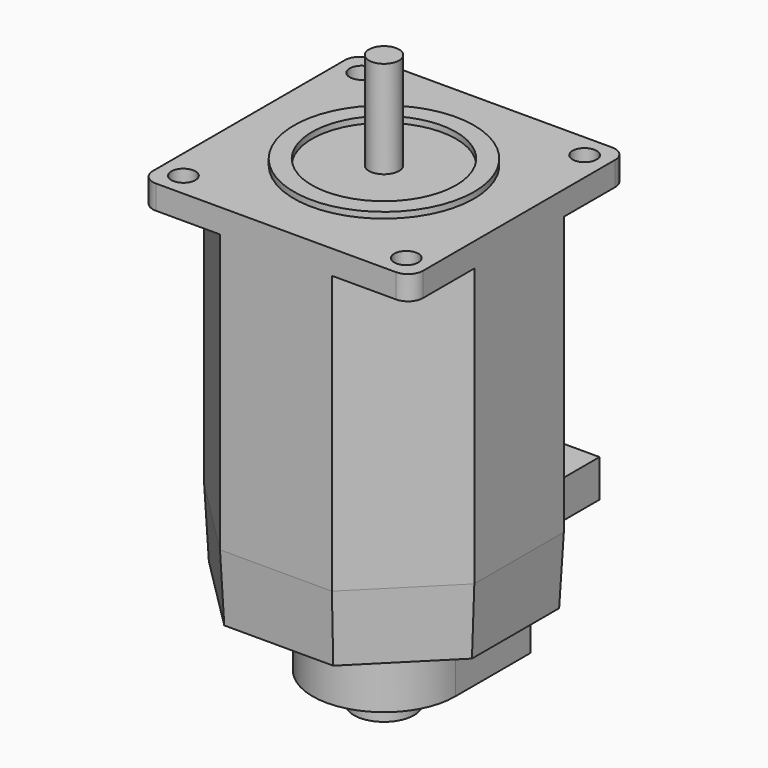
from build123d import *

# Parameters (mm, degrees)
F0_R                   = 2.54
F0_R_2                 = 19.05
F0_R_3                 = 15.24
F0_R_4                 = 3.175
F1_DEPTH               = 5.08
F2_DEPTH               = 1.27
F3_DEPTH               = 20.574
F5_DEPTH               = 58.7375
F6_DEPTH               = 14.2875
DRAFT_F6_DRAFTED_ANGLE = 3
F7_R                   = 6.35
F8_DEPTH               = 22.225
F9_DEPTH               = 15.875
F11_DEPTH              = 3.175
F12_DEPTH              = 12.7
F13_T                  = 1.27
F13_T3_DEPTH           = 26.2123050896
F13_T5_DEPTH           = 3.9232108179
F13_T7_DEPTH           = 10.4992710847
F13_T9_DEPTH           = 3.6795314226
F13_T11_DEPTH          = 26.0744592074
F13_T13_DEPTH          = 3.6795314226
F13_T15_DEPTH          = 10.4992710847
F13_T17_DEPTH          = 3.9232108179
F13_T19_DEPTH          = 26.2123050896
F13_T21_DEPTH          = 25.7298445017
F13_T23_DEPTH          = 22.38375
F13_T25_DEPTH          = 32.7025
F13_T27_DEPTH          = 26.2123050896
F13_T29_DEPTH          = 26.2123050896
F13_T34_ANGLE          = 180.000000001


# Not quite as in the source:
# - an extrude with a draft is written as a straight extrude whose walls are then drafted
# - a shell that OpenCascade refuses in one call is made with other operations: the cavity is built on its own and cut out


with BuildPart() as f1:
    # F0 (on Top) → F1 (new body)
    with BuildSketch(Plane.XY):
        with BuildLine():
            Line((-53.975, 0), (-3.175, 0))
            ThreePointArc((-3.175, 0), (-0.9299359697, 0.9299359697), (0, 3.175))
            Line((0, 3.175), (0, 53.975))
            ThreePointArc((0, 53.975), (-0.9299359697, 56.2200640303), (-3.175, 57.15))
            Line((-3.175, 57.15), (-53.975, 57.15))
            ThreePointArc((-53.975, 57.15), (-56.2200640303, 56.2200640303), (-57.15, 53.975))
            Line((-57.15, 53.975), (-57.15, 3.175))
            ThreePointArc((-57.15, 3.175), (-56.2200640303, 0.9299359697), (-53.975, 0))
        make_face()
        with Locations((-52.1481723178, 5.0018276822)):
            Circle(F0_R, mode=Mode.SUBTRACT)
        with Locations((-5.0018276822, 5.0018276822)):
            Circle(F0_R, mode=Mode.SUBTRACT)
        with Locations((-52.1481723178, 52.1481723178)):
            Circle(F0_R, mode=Mode.SUBTRACT)
        with Locations((-28.575, 28.575)):
            Circle(F0_R_2, mode=Mode.SUBTRACT)
        with Locations((-5.0018276822, 52.1481723178)):
            Circle(F0_R, mode=Mode.SUBTRACT)
        with Locations((-28.575, 28.575)):
            Circle(F0_R_2)
        with Locations((-28.575, 28.575)):
            Circle(F0_R_3, mode=Mode.SUBTRACT)
        with Locations((-28.575, 28.575)):
            Circle(F0_R_3)
        with Locations((-28.575, 28.575)):
            Circle(F0_R_4, mode=Mode.SUBTRACT)
        with Locations((-28.575, 28.575)):
            Circle(F0_R_4)
    extrude(amount=-F1_DEPTH)

    # F0 (on Top) → F2 (join)
    with BuildSketch(Plane.XY):
        with Locations((-28.575, 28.575)):
            Circle(F0_R_2)
        with Locations((-28.575, 28.575)):
            Circle(F0_R_3, mode=Mode.SUBTRACT)
    extrude(amount=F2_DEPTH)

    # F0 (on Top) → F3 (join)
    with BuildSketch(Plane.XY):
        with Locations((-28.575, 28.575)):
            Circle(F0_R_4)
    extrude(amount=F3_DEPTH)

    # F4 (on face) → F5 (join)
    with BuildSketch(Plane(origin=(0, 0, -5.08), x_dir=(1, 0, 0), z_dir=(0, 0, -1))):
        Polygon((-40.4111525448, -57.15), (-16.7388474552, -57.15), (0, -40.4111525448), (0, -16.7388474552), (-16.7388474552, 0), (-40.4111525448, 0), (-57.15, -16.7388474552), (-57.15, -40.4111525448), align=None)
    extrude(amount=F5_DEPTH)


with BuildPart() as f6_drafted:
    # F6 (new): a face of the model
    f6_faces = [f1.part.faces().sort_by_distance(p)[0] for p in [
        (-28.575, 28.575, -63.8175),
    ]]
    extrude(f6_faces, amount=F6_DEPTH)

    # draft_F6_drafted
    draft_f6_drafted_walls = [f6_drafted.faces().sort_by_distance(p)[0] for p in [
        (-28.575, 57.15, -73.3425),
        (-8.3694237276, 48.7805762724, -73.3425),
        (0, 28.575, -73.3425),
        (-8.3694237276, 8.3694237276, -73.3425),
        (-28.575, 0, -73.3425),
        (-48.7805762724, 8.3694237276, -73.3425),
        (-57.15, 28.575, -73.3425),
        (-48.7805762724, 48.7805762724, -73.3425),
    ]]
    draft(draft_f6_drafted_walls, neutral_plane=Plane(origin=(-28.575, 28.575, -63.8175), x_dir=(1, 0, 0), z_dir=(0, 0, -1)), angle=DRAFT_F6_DRAFTED_ANGLE)


with BuildPart() as f1_1:
    add(f1.part)

    # join_F6_drafted: union F6_drafted
    add(f6_drafted.part)

    # F7 (on face) → F8 (join)
    with BuildSketch(Plane(origin=(0, 0, -78.105), x_dir=(1, 0, 0), z_dir=(0, 0, -1))):
        with Locations((-28.575, -28.575)):
            Circle(F7_R)
    extrude(amount=F8_DEPTH)

    # F7 (on face) → F9 (join)
    with BuildSketch(Plane(origin=(0, 0, -78.105), x_dir=(1, 0, 0), z_dir=(0, 0, -1))):
        with BuildLine():
            Line((-13.49375, -48.41875), (-13.49375, -28.575))
            ThreePointArc((-13.49375, -28.575), (-28.575, -13.49375), (-43.65625, -28.575))
            Line((-43.65625, -28.575), (-43.65625, -48.41875))
            Line((-43.65625, -48.41875), (-13.49375, -48.41875))
        make_face()
        with Locations((-28.575, -28.575)):
            Circle(F7_R, mode=Mode.SUBTRACT)
    extrude(amount=F9_DEPTH)

    # F10 (on face) → F11 (join)
    with BuildSketch(Plane(origin=(0, 57.15, 0), x_dir=(-1, 0, 0), z_dir=(0, 1, 0))):
        Polygon((16.002, -74.93), (28.575, -74.93), (41.148, -74.93), (41.148, -66.9925), (16.002, -66.9925), align=None)
    extrude(amount=-F11_DEPTH)

    # F12 (add): a face of the model
    f12_faces = [f1_1.faces().sort_by_distance(p)[0] for p in [
        (-28.575, 57.15, -70.96125),
    ]]
    extrude(f12_faces, amount=F12_DEPTH)

    # F13: shell of thickness 1.27, made by hand


with BuildPart() as f13_core1:
    # F13_t2: copy of F1
    add(f1_1.part)

    # the walls: a layer under each face that stays
    f13_faces = [f13_core1.faces().sort_by_distance(p)[0] for p in [
        (-28.575, 0, -31.90875),
        (-47.625, 9.525, 0),
        (-7.5418276822, 52.1481723178, -2.54),
        (-8.3694237276, 54.3601920908, -5.08),
        (-8.3694237276, 48.7805762724, -34.44875),
        (-8.634156073, 48.515843927, -70.96125),
        (-28.575, 57.0668026504, -65.405),
        (-48.515843927, 48.515843927, -70.96125),
        (-56.7756119267, 28.575, -70.96125),
        (-48.515843927, 8.634156073, -70.96125),
        (-41.148, 62.7197704018, -70.96125),
        (-48.7805762724, 48.7805762724, -34.44875),
        (-54.3601920908, 48.7805762724, -5.08),
        (-28.575, 63.0139174522, -66.9925),
        (-16.002, 62.7197704018, -70.96125),
        (-28.575, 62.7197704018, -74.93),
        (-28.575, 56.4844212031, -76.5175),
        (-47.1258159023, 47.1258159023, -78.105),
        (-28.575, 13.49375, -86.0425),
        (-38.6291666667, 42.5979166667, -93.98),
        (-34.925, 28.575, -97.155),
        (-28.575, 28.575, -100.33),
        (-13.49375, 38.496875, -86.0425),
        (-28.575, 48.41875, -86.0425),
        (-43.65625, 38.496875, -86.0425),
        (-8.634156073, 8.634156073, -70.96125),
        (-0.3743880733, 28.575, -70.96125),
        (-54.6881723178, 52.1481723178, -2.54),
        (-47.625, 28.575, 0.635),
        (-41.275, 15.875, 1.27),
        (-43.815, 28.575, 0.635),
        (-38.735, 18.415, 0),
        (-31.75, 28.575, 10.287),
        (-28.575, 28.575, 20.574),
        (-7.5418276822, 5.0018276822, -2.54),
        (-54.6881723178, 5.0018276822, -2.54),
        (-28.575, 57.15, -31.90875),
        (-0.9299359697, 56.2200640303, -2.54),
        (-56.2200640303, 56.2200640303, -2.54),
        (0, 28.575, -31.90875),
        (-57.15, 28.575, -31.90875),
        (-0.9299359697, 0.9299359697, -2.54),
        (-8.3694237276, 2.7898079092, -5.08),
        (-8.3694237276, 8.3694237276, -34.44875),
        (-28.575, 0.3743880733, -70.96125),
        (-48.7805762724, 8.3694237276, -34.44875),
        (-54.3601920908, 2.7898079092, -5.08),
        (-56.2200640303, 0.9299359697, -2.54),
    ]]
    thicken(f13_faces, amount=-F13_T, mode=Mode.SUBTRACT)

    # F13_s4 → F13_t3 (cut)
    with BuildSketch(Plane(origin=(-37.8424493397, 37.8424493397, 0), x_dir=(0, 0, 1), z_dir=(0.7071067812, -0.7071067812, 0))):
        Polygon((-5.0927, -28.5877), (-3.81, -28.575), (-3.81, -27.305), (-5.08, -27.305), align=None)
    extrude(amount=F13_T3_DEPTH, mode=Mode.SUBTRACT)

    # F13_s6 → F13_t5 (cut)
    with BuildSketch(Plane(origin=(-37.671873763, 37.671873763, 0), x_dir=(0, 0, 1), z_dir=(0.7071067812, -0.7071067812, 0))):
        Polygon((-74.9433646666, -28.0053011478), (-74.8635333356, -26.7243590436), (-73.66, -26.787433553), (-73.66, -27.9926185527), align=None)
    extrude(amount=F13_T5_DEPTH, mode=Mode.SUBTRACT)

    # F13_s8 → F13_t7 (cut)
    with BuildSketch(Plane(origin=(0, -5.3133328807, -71.689618641), x_dir=(1, 0, 0), z_dir=(0, 0.0739130625, 0.9972646886))):
        Polygon((-15.980332051, 60.9847844179), (-16.8987948992, 60.0765372308), (-17.272, 60.4487214994), (-17.272, 60.9757918715), align=None)
    extrude(amount=F13_T7_DEPTH, mode=Mode.SUBTRACT)

    # F13_s10 → F13_t9 (cut)
    with BuildSketch(Plane(origin=(-35.1918918401, 35.1918918401, 0), x_dir=(0, 0, 1), z_dir=(-0.7071067812, 0.7071067812, 0))):
        Polygon((-66.9804646666, 28.4212878959), (-66.9260333356, 27.1403457916), (-68.2625, 27.0703045417), (-68.2625, 28.4086053008), align=None)
    extrude(amount=F13_T9_DEPTH, mode=Mode.SUBTRACT)

    # F13_s12 → F13_t11 (cut)
    with BuildSketch(Plane.YZ.offset(-41.6122296037)):
        Polygon((56.9962878959, -66.9804646666), (55.7153457916, -66.9260333356), (55.6453045417, -68.2625), (56.9836053008, -68.2625), align=None)
    extrude(amount=F13_T11_DEPTH, mode=Mode.SUBTRACT)

    # F13_s14 → F13_t13 (cut)
    with BuildSketch(Plane(origin=(9.2187134607, 9.2187134607, 0), x_dir=(0, 0, 1), z_dir=(-0.7071067812, -0.7071067812, 0))):
        Polygon((-66.9804646666, 68.8324404407), (-66.9260333356, 67.5514983364), (-68.2625, 67.4814570865), (-68.2625, 68.8197578456), align=None)
    extrude(amount=F13_T13_DEPTH, mode=Mode.SUBTRACT)

    # F13_s16 → F13_t15 (cut)
    with BuildSketch(Plane(origin=(0, -4.5372996011, -61.2190663319), x_dir=(1, 0, 0), z_dir=(0, -0.0739130625, -0.9972646886))):
        Polygon((-41.169667949, -60.9847844179), (-40.2512051008, -60.0765372308), (-39.878, -60.4487214994), (-39.878, -60.9757918715), align=None)
    extrude(amount=F13_T15_DEPTH, mode=Mode.SUBTRACT)

    # F13_s18 → F13_t17 (cut)
    with BuildSketch(Plane(origin=(6.3227447897, 6.3227447897, 0), x_dir=(0, 0, 1), z_dir=(0.7071067812, 0.7071067812, 0))):
        Polygon((-74.9433646666, -68.4164536926), (-74.8635333356, -67.1355115884), (-73.66, -67.1985860978), (-73.66, -68.4037710975), align=None)
    extrude(amount=F13_T17_DEPTH, mode=Mode.SUBTRACT)

    # F13_s20 → F13_t19 (cut)
    with BuildSketch(Plane(origin=(-9.2674493397, -9.2674493397, 0), x_dir=(0, 0, 1), z_dir=(0.7071067812, 0.7071067812, 0))):
        Polygon((-5.0927, -68.9988525448), (-5.08, -67.7161525448), (-3.81, -67.7161525448), (-3.81, -68.9861525448), align=None)
    extrude(amount=F13_T19_DEPTH, mode=Mode.SUBTRACT)

    # F13_s22 → F13_t21 (cut)
    with BuildSketch(Plane.YZ.offset(-41.4399222509)):
        Polygon((56.5803011478, -74.9433646666), (56.5676185527, -73.66), (55.362433553, -73.66), (55.2993590436, -74.8635333356), align=None)
    extrude(amount=F13_T21_DEPTH, mode=Mode.SUBTRACT)

    # F13_s24 → F13_t23 (cut)
    with BuildSketch(Plane.XZ.offset(-49.68875)):
        Polygon((-43.66895, -78.1177), (-43.65625, -76.835), (-42.38625, -76.835), (-42.38625, -78.105), align=None)
        Polygon((-13.48105, -78.1177), (-13.49375, -76.835), (-14.76375, -76.835), (-14.76375, -78.105), align=None)
    extrude(amount=F13_T23_DEPTH, mode=Mode.SUBTRACT)

    # F13_s26 → F13_t25 (cut)
    with BuildSketch(Plane.YZ.offset(-44.92625)):
        Polygon((48.43145, -78.1177), (48.41875, -76.835), (47.14875, -76.835), (47.14875, -78.105), align=None)
    extrude(amount=F13_T25_DEPTH, mode=Mode.SUBTRACT)

    # F13_s28 → F13_t27 (cut)
    with BuildSketch(Plane(origin=(9.2674493397, 9.2674493397, 0), x_dir=(0, 0, 1), z_dir=(-0.7071067812, -0.7071067812, 0))):
        Polygon((-5.0927, 11.8234525448), (-3.81, 11.8361525448), (-3.81, 13.1061525448), (-5.08, 13.1061525448), align=None)
    extrude(amount=F13_T27_DEPTH, mode=Mode.SUBTRACT)

    # F13_s30 → F13_t29 (cut)
    with BuildSketch(Plane(origin=(-19.3075506603, 19.3075506603, 0), x_dir=(0, 0, 1), z_dir=(-0.7071067812, 0.7071067812, 0))):
        Polygon((-5.0927, -28.5877), (-5.08, -27.305), (-3.81, -27.305), (-3.81, -28.575), align=None)
    extrude(amount=F13_T29_DEPTH, mode=Mode.SUBTRACT)

    # F13_s31 → F13_t32 (revolve, cut)
    with BuildSketch(Plane.XZ.offset(-28.575)):
        Polygon((-9.5123, 0.0127), (-9.525, -1.27), (-10.795, -1.27), (-10.795, 0), align=None)
    revolve(axis=Axis((-28.575, 28.575, 0), (0, 0, 1)), mode=Mode.SUBTRACT)

    # F13_s33 → F13_t34 (revolve, cut)
    with BuildSketch(Plane.XZ.offset(-28.575)):
        Polygon((-13.48105, -78.1177), (-13.49375, -76.835), (-14.76375, -76.835), (-14.76375, -78.105), align=None)
    revolve(axis=Axis((-28.575, 28.575, -78.105), (0, 0, -1)), revolution_arc=F13_T34_ANGLE, mode=Mode.SUBTRACT)

    # F13_s35 → F13_t36 (revolve, cut)
    with BuildSketch(Plane.XZ.offset(-28.575)):
        Polygon((-22.2123, -93.9927), (-22.225, -92.71), (-23.495, -92.71), (-23.495, -93.98), align=None)
    revolve(axis=Axis((-28.575, 28.575, -93.98), (0, 0, -1)), mode=Mode.SUBTRACT)

    # F13_s37 → F13_t38 (revolve, cut)
    with BuildSketch(Plane.XZ.offset(-28.575)):
        Polygon((-13.3477, 0.0127), (-12.065, 0), (-12.065, -1.27), (-13.335, -1.27), align=None)
    revolve(axis=Axis((-28.575, 28.575, 0), (0, 0, 1)), mode=Mode.SUBTRACT)

    # F13_s39 → F13_t40 (revolve, cut)
    with BuildSketch(Plane.XZ.offset(-28.575)):
        Polygon((-25.3873, 0.0127), (-25.4, -1.27), (-26.67, -1.27), (-26.67, 0), align=None)
    revolve(axis=Axis((-28.575, 28.575, 0), (0, 0, 1)), mode=Mode.SUBTRACT)


with BuildPart() as f1_2:
    add(f1_1.part)

    # what is left inside the walls is the cavity
    f13_cavity = [f13_core1.part.solids().sort_by_distance(p)[0] for p in [
        (-54.851229, 2.298771, -2.963333),
        (-14.9225, 7.337778, -1.2827),
        (-2.298771, 2.298771, -2.963333),
        (-2.298771, 54.851229, -2.963333),
        (-54.851229, 54.851229, -2.963333),
    ]]
    add(f13_cavity, mode=Mode.SUBTRACT)


solid = f1_2.part
